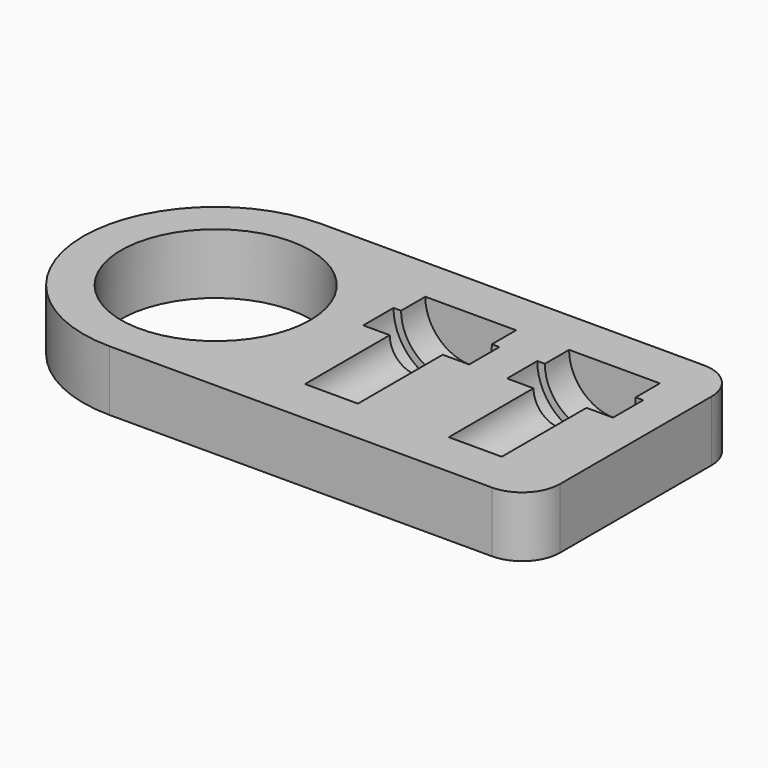
from build123d import *

# Parameters (mm, degrees)
F0_R         = 12.5
F1_DEPTH     = 8
F5_TEXT_SIZE = 5.5555555556
F6_DEPTH     = 1


# Not quite as in the source:
# - Text() gives the source's letters only with a copy of the font that has no kerning and outlines rounded to 1/6400 em; it was checked with that copy


with BuildPart() as f1:
    # F0 (on Top) → F1 (new body)
    with BuildSketch(Plane.XY):
        with BuildLine():
            ThreePointArc((0, 17.5), (5.1256313292, 5.1256313292), (17.5, 0))
            Line((17.5, 0), (68, 0))
            ThreePointArc((68, 0), (71.5355339059, 1.4644660941), (73, 5))
            Line((73, 5), (73, 30))
            ThreePointArc((73, 30), (71.5355339059, 33.5355339059), (68, 35))
            Line((68, 35), (17.5, 35))
            ThreePointArc((17.5, 35), (5.1256313292, 29.8743686708), (0, 17.5))
        make_face()
        with Locations((17.5, 17.5)):
            Circle(F0_R, mode=Mode.SUBTRACT)
    extrude(amount=F1_DEPTH)

    # F2 (on face) → F3 (revolve, cut)
    with BuildSketch(Plane.XY.offset(8)):
        Polygon((42, 20), (42, 6), (45.5, 6), (45.5, 20), (49, 20), (49, 25), (48, 25), (48, 29), (42, 29), (42, 25), align=None)
    revolve(axis=Axis((42, 22.5, 8), (0, 1, 0)), mode=Mode.SUBTRACT)

    # F2 (on face) → F4 (revolve, cut)
    with BuildSketch(Plane.XY.offset(8)):
        Polygon((61, 20), (61, 6), (64.5, 6), (64.5, 20), (68, 20), (68, 25), (67, 25), (67, 29), (61, 29), (61, 25), align=None)
    revolve(axis=Axis((61, 22.5, 8), (0, 1, 0)), mode=Mode.SUBTRACT)

    # F5 (on face) → F6 (cut)
    with BuildSketch(Plane(origin=(0, 0, 0), x_dir=(1, 0, 0), z_dir=(0, 0, -1))):
        with Locations((30, -9)):
            Text('833, 871', F5_TEXT_SIZE, font='Open Sans', text_align=(TextAlign.LEFT, TextAlign.BOTTOM))
    extrude(amount=-F6_DEPTH, mode=Mode.SUBTRACT)


solid = f1.part
